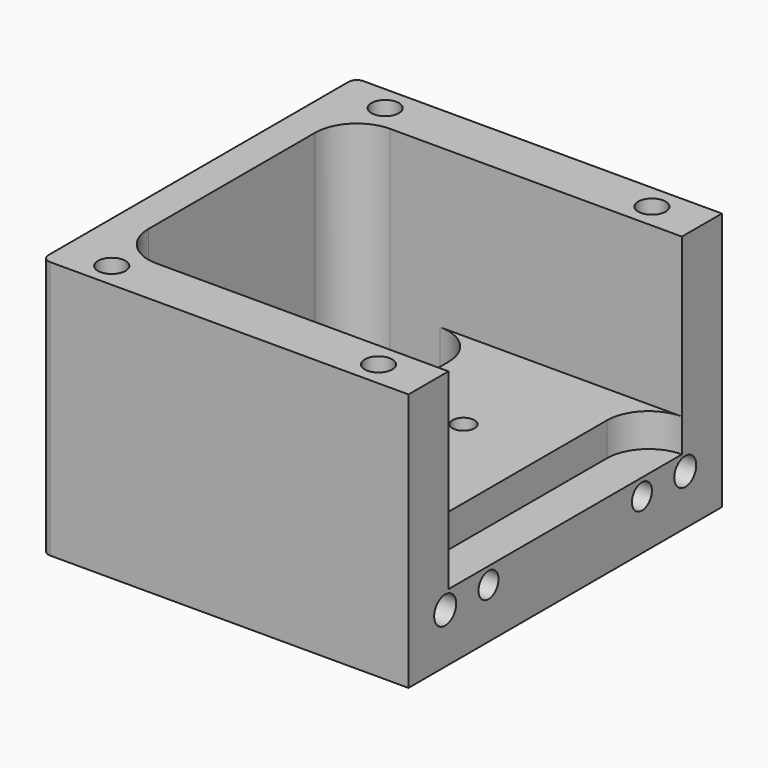
from build123d import *

# Parameters (mm, degrees)
F1_DEPTH  = 31
F3_DEPTH  = 19
F5_DEPTH  = 8
F8_D      = 3.3
F8_DEPTH  = 10
F8_TIP    = 0.9914200214
F9_DEPTH  = 4
F11_D     = 2.65
F11_DEPTH = 10
F11_TIP   = 0.7961403202
F13_D     = 3
F13_DEPTH = 10
F13_TIP   = 0.9012909285
F14_D     = 3.3
F14_DEPTH = 10
F14_TIP   = 0.9914200214
F15_R     = 1


# Not quite as in the source:
# - ends of sketch curves that miss each other by under 0.0002 mm in the source are joined


with BuildPart() as f1:
    # F0 (on Top) → F1 (new body)
    with BuildSketch(Plane.XY):
        Polygon((-27, -28.75), (0, -28.75), (17, -28.75), (17, 18.25), (-27, 18.25), align=None)
    extrude(amount=F1_DEPTH)

    # F2 (on face) → F3 (cut)
    with BuildSketch(Plane.XY.offset(31)):
        with BuildLine():
            Line((17, -22.75), (17, 12.25))
            Line((17, 12.25), (-18, 12.25))
            ThreePointArc((-18, 12.25), (-21.5355339059, 10.7855339059), (-23, 7.25))
            Line((-23, 7.25), (-23, -17.75))
            ThreePointArc((-23, -17.75), (-21.5355339059, -21.2855339059), (-18, -22.75))
            Line((-18, -22.75), (17, -22.75))
        make_face()
    extrude(amount=-F3_DEPTH, mode=Mode.SUBTRACT)

    # F4 (on face) → F5 (cut)
    with BuildSketch(Plane.XY.offset(12)):
        with BuildLine():
            Line((-7, -17.7601174265), (-7, -5.25))
            Line((-7, -5.25), (-7, 7.25))
            ThreePointArc((-7, 7.25), (-8.4644660941, 10.7855339059), (-12, 12.25))
            Line((-12, 12.25), (-18, 12.25))
            ThreePointArc((-18, 12.25), (-21.5355339059, 10.7855339059), (-23, 7.25))
            Line((-23, 7.25), (-23, -17.75))
            Line((-23, -17.75), (-23, -17.7601174265))
            ThreePointArc((-23, -17.7601174265), (-21.5319550515, -21.2891091414), (-18, -22.75))
            Line((-18, -22.75), (-11.6820819243, -22.75))
            ThreePointArc((-11.6820819243, -22.75), (-8.3537971547, -21.1814044374), (-7, -17.7601174265))
        make_face()
    extrude(amount=-F5_DEPTH, mode=Mode.SUBTRACT)

    # F8
    with Locations(Plane.XY.offset(31)):
        with Locations((-21, 15.25), (-21, -25.75), (11, -25.75), (11, 15.25)):
            Hole(F8_D / 2, depth=F8_DEPTH)
            with Locations((0, 0, -(F8_DEPTH + F8_TIP / 2))):  # 118° drill point
                Cone(0, F8_D / 2, F8_TIP, mode=Mode.SUBTRACT)

    # F6 (on face) → F9 (cut)
    with BuildSketch(Plane.XY.offset(12)):
        with BuildLine():
            Line((17, -22.75), (17, 12.25))
            ThreePointArc((17, 12.25), (13.4644660941, 10.7855339059), (12, 7.25))
            Line((12, 7.25), (12, -17.75))
            ThreePointArc((12, -17.75), (13.4644660941, -21.2855339059), (17, -22.75))
        make_face()
    extrude(amount=-F9_DEPTH, mode=Mode.SUBTRACT)

    # F11
    with Locations(Plane.XY.offset(12)):
        with Locations((2, -1.75), (2, -8.75)):
            Hole(F11_D / 2, depth=F11_DEPTH)
            with Locations((0, 0, -(F11_DEPTH + F11_TIP / 2))):  # 118° drill point
                Cone(0, F11_D / 2, F11_TIP, mode=Mode.SUBTRACT)

    # F13
    with Locations(Plane.YZ.offset(17)):
        with Locations((-16.75, 6), (6.25, 6)):
            Hole(F13_D / 2, depth=F13_DEPTH)
            with Locations((0, 0, -(F13_DEPTH + F13_TIP / 2))):  # 118° drill point
                Cone(0, F13_D / 2, F13_TIP, mode=Mode.SUBTRACT)

    # F14
    with Locations(Plane.YZ.offset(17)):
        with Locations((12.75, 6), (-23.25, 6)):
            Hole(F14_D / 2, depth=F14_DEPTH)
            with Locations((0, 0, -(F14_DEPTH + F14_TIP / 2))):  # 118° drill point
                Cone(0, F14_D / 2, F14_TIP, mode=Mode.SUBTRACT)

    # F15
    f15_edges = [f1.edges().sort_by_distance(p)[0] for p in [
        (-27, -28.75, 15.5),
        (-27, 18.25, 15.5),
    ]]
    fillet(f15_edges, radius=F15_R)


solid = f1.part
